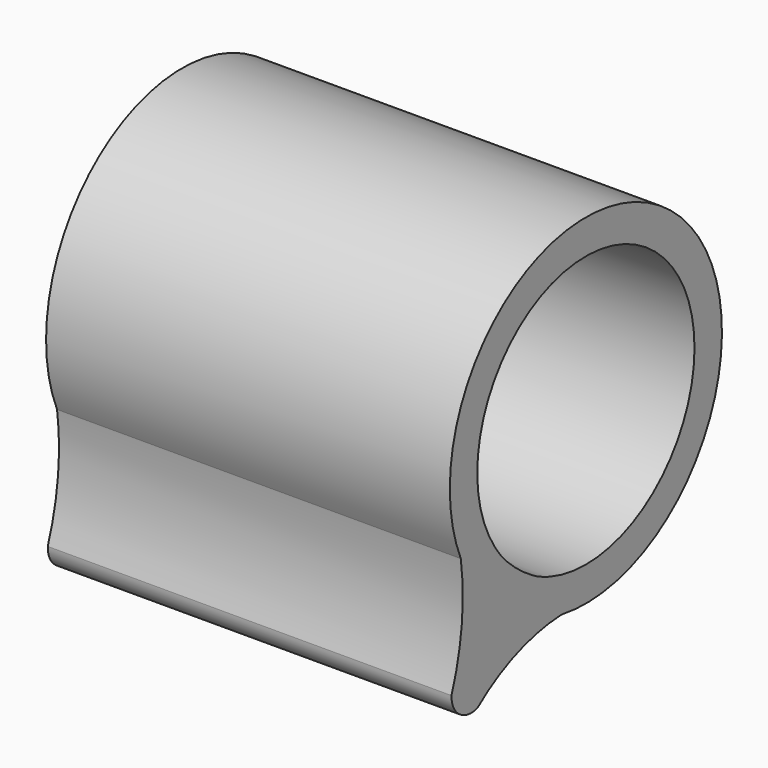
from build123d import *

# Parameters (mm, degrees)
F0_R     = 4.2799
F1_DEPTH = 8.89
F2_DEPTH = 10.16
F3_DEPTH = 8.89
F5_DEPTH = 9.779
F7_DEPTH = 10.16


# Not quite as in the source:
# - a feature names something its author has since deleted; it is built from what else it names


with BuildPart() as f1:
    # F0 (on Right) → F1 (new body)
    with BuildSketch(Plane.YZ):
        Circle(F0_R)
        with BuildLine():
            ThreePointArc((-2.5770476719, -2.2427507634), (-1.1973173615, 3.1996151059), (3.4163, 0))
            ThreePointArc((3.4163, 0), (1.7788031507, -2.9166701975), (-1.563921316, -3.0373106208))
            ThreePointArc((-1.563921316, -3.0373106208), (-2.1082545817, -2.6881905268), (-2.5770476719, -2.2427507634))
        make_face(mode=Mode.SUBTRACT)
        with BuildLine():
            ThreePointArc((-1.563921316, -3.0373106208), (-1.8240626008, -2.3258233831), (-2.5770476719, -2.2427507634))
            ThreePointArc((-2.5770476719, -2.2427507634), (-2.1082545817, -2.6881905268), (-1.563921316, -3.0373106208))
        make_face()
    extrude(amount=F1_DEPTH)

    # F2 (add): a face of the model
    f2_faces = [f1.faces().sort_by_distance(p)[0] for p in [
        (8.89, -4.1588461475, 0),
    ]]
    extrude(f2_faces, amount=F2_DEPTH)

    # F3 (cut): a face of the model
    f3_faces = [f1.faces().sort_by_distance(p)[0] for p in [
        (0, -4.1588461475, 0),
    ]]
    extrude(f3_faces, amount=-F3_DEPTH, mode=Mode.SUBTRACT)

    # F4 (on face) → F5 (cut)
    with BuildSketch(Plane.YZ.offset(19.05)):
        with BuildLine():
            ThreePointArc((1.222316808, 3.1901484779), (-2.6598297691, 2.1439242733), (-2.8578464427, -1.8718491926))
            ThreePointArc((-2.8578464427, -1.8718491926), (-2.7221442185, -2.0613321722), (-2.5741425301, -2.2413721494))
            ThreePointArc((-2.5741425301, -2.2413721494), (-1.8240626008, -2.3258233831), (-1.5632748259, -3.0341606246))
            ThreePointArc((-1.5632748259, -3.0341606246), (-1.3531490958, -3.134987559), (-1.1367838725, -3.2216188659))
            ThreePointArc((-1.1367838725, -3.2216188659), (2.6552480052, -2.1495961762), (2.9143968144, 1.7825254271))
            ThreePointArc((2.9143968144, 1.7825254271), (2.1811855738, 2.6219665113), (1.222316808, 3.1901484779))
        make_face()
        with BuildLine():
            ThreePointArc((-1.5632748259, -3.0341606246), (-1.8240626008, -2.3258233831), (-2.5741425301, -2.2413721494))
            ThreePointArc((-2.5741425301, -2.2413721494), (-2.5391071094, -2.2806143375), (-2.5034863371, -2.3193259716))
            ThreePointArc((-2.5034863371, -2.3193259716), (-2.1009284684, -2.6788491558), (-1.6558220878, -2.9841196383))
            ThreePointArc((-1.6558220878, -2.9841196383), (-1.6097363346, -3.009487598), (-1.5632748259, -3.0341606246))
        make_face()
    extrude(amount=-F5_DEPTH, mode=Mode.SUBTRACT)

    # F6 (on face) → F7 (join)
    with BuildSketch(Plane.YZ.offset(19.05)):
        with BuildLine():
            Line((-3.4094376469, -5.2050021479), (-3.808154026, -4.9026301131))
            Line((-3.808154026, -4.9026301131), (-4.2274528535, -4.5974798009))
            ThreePointArc((-4.2274528535, -4.5974798009), (-3.9771826251, -5.1149772874), (-3.4094376469, -5.2050021479))
        make_face()
        with BuildLine():
            ThreePointArc((-0.7629935409, -4.2113400322), (-1.5232386045, -3.9996610061), (-2.2316948802, -3.6519969841))
            Line((-2.2316948802, -3.6519969841), (-3.4094376469, -5.2050021479))
            ThreePointArc((-3.4094376469, -5.2050021479), (-2.1650447738, -4.4982234477), (-0.7629935409, -4.2113400322))
        make_face()
        with BuildLine():
            Line((-4.2274528535, -4.5974798009), (-3.0318107196, -3.0208720215))
            ThreePointArc((-3.0318107196, -3.0208720215), (-3.5466345046, -2.3956059152), (-3.9344436304, -1.6845466242))
            ThreePointArc((-3.9344436304, -1.6845466242), (-3.9036835411, -3.1588441029), (-4.2274528535, -4.5974798009))
        make_face()
        with BuildLine():
            Line((-2.6242534582, -3.3423499234), (-2.6430441595, -3.3662830512))
            ThreePointArc((-2.6430441595, -3.3662830512), (-2.4415524342, -3.515162261), (-2.2316948802, -3.6519969841))
            Line((-2.2316948802, -3.6519969841), (-2.6242534582, -3.3423499234))
        make_face()
        with BuildLine():
            ThreePointArc((-3.0318107196, -3.0208720215), (-2.8426786082, -3.1994878247), (-2.6430441595, -3.3662830512))
            Line((-2.6430441595, -3.3662830512), (-2.6242534582, -3.3423499234))
            Line((-2.6242534582, -3.3423499234), (-3.0318107196, -3.0208720215))
        make_face()
        with BuildLine():
            ThreePointArc((-2.2316948802, -3.6519969841), (-2.4415524342, -3.515162261), (-2.6430441595, -3.3662830512))
            Line((-2.6430441595, -3.3662830512), (-3.808154026, -4.9026301131))
            Line((-3.808154026, -4.9026301131), (-3.4094376469, -5.2050021479))
            Line((-3.4094376469, -5.2050021479), (-2.2316948802, -3.6519969841))
        make_face()
        with BuildLine():
            Line((-3.808154026, -4.9026301131), (-2.6430441595, -3.3662830512))
            ThreePointArc((-2.6430441595, -3.3662830512), (-2.8426786082, -3.1994878247), (-3.0318107196, -3.0208720215))
            Line((-3.0318107196, -3.0208720215), (-4.2274528535, -4.5974798009))
            Line((-4.2274528535, -4.5974798009), (-3.808154026, -4.9026301131))
        make_face()
    extrude(amount=-F7_DEPTH)


solid = f1.part
